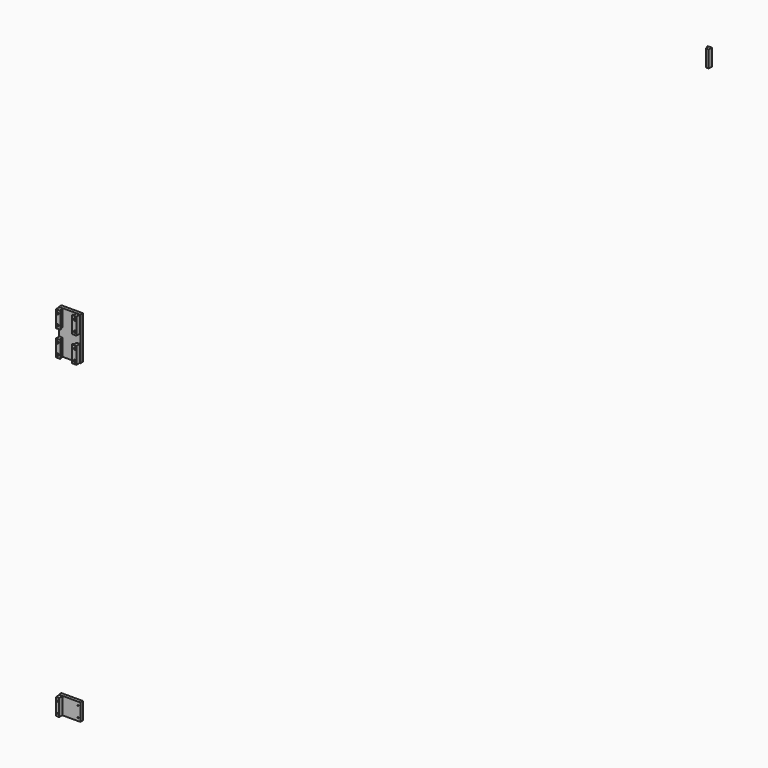
from build123d import *

# Parameters (mm, degrees)
F1_W           = 100
F1_H           = 200
F2_DEPTH       = 15
F3_D           = 5
F4_W           = 15
F4_H           = 78
F4_R           = 2.5
F5_DEPTH       = 20
F7_D           = 6.6
F7_CBORE_D     = 11.25
F7_CBORE_DEPTH = 6
F8_W           = 5
F8_H           = 78
F9_DEPTH       = 5
F10_W          = 100
F10_H          = 80
F11_DEPTH      = 15
F12_W          = 15
F12_H          = 78
F13_DEPTH      = 20
F15_D          = 5
F15_2_D        = 5
F23_DEPTH      = 78


# Not quite as in the source:
# - a pattern or mirror of a feature is missing from the dataset's text; its kind, count and spacing are read off the source's solid


with BuildPart() as f2:
    # F1 (on Front) → F2 (new body)
    with BuildSketch(Plane.XZ):
        with Locations((-2997.1325380377, -2081.9933028066)):
            Rectangle(F1_W, F1_H)
    extrude(amount=F2_DEPTH)

    # F3 (through all)
    with Locations(Plane(origin=(0, 0, 0), x_dir=(1, 0, 0), z_dir=(0, 1, 0))):
        with Locations((-3037.6325380377, 1996.9933028066), (-2956.6325380377, 1996.9933028066), (-2956.6325380377, 2046.9933028066), (-3037.6325380377, 2046.9933028066), (-3037.6325380377, 2116.9933028066), (-2956.6325380377, 2116.9933028066), (-3037.6325380377, 2166.9933028066), (-2956.6325380377, 2166.9933028066)):
            Hole(F3_D / 2)


with BuildPart() as f5:
    # F4 (on face) → F5 (new body)
    with BuildSketch(Plane.XZ.offset(15)):
        with Locations((-3037.1325380377, -2021.9933028066)):
            Rectangle(F4_W, F4_H)
        with Locations((-3037.6325380377, -2046.9933028066)):
            Circle(F4_R, mode=Mode.SUBTRACT)
        with Locations((-3037.6325380377, -1996.9933028066)):
            Circle(F4_R, mode=Mode.SUBTRACT)
    extrude(amount=F5_DEPTH)

    # F7 (through all)
    with Locations(Plane.XZ.offset(35)):
        with Locations((-3037.6325380377, -1996.9933028066), (-3037.6325380377, -2046.9933028066)):
            CounterBoreHole(F7_D / 2, F7_CBORE_D / 2, F7_CBORE_DEPTH)

    # F8 (on face) → F9 (join)
    with BuildSketch(Plane.YZ.offset(-3029.6325380377)):
        with Locations((-32.5, -2021.9933028066)):
            Rectangle(F8_W, F8_H)
    extrude(amount=F9_DEPTH)


with BuildPart() as f11:
    # F10 (on face) → F11 (new body)
    with BuildSketch(Plane.XZ):
        with Locations((-2997.1325380377, -3614.9933028066)):
            Rectangle(F10_W, F10_H)
    extrude(amount=F11_DEPTH)

    # F15 (through all)
    with Locations(Plane.XZ.offset(35)):
        with Locations((-3037.1325380377, -3590.9933028066), (-3037.1325380377, -3640.9933028066)):
            f15 = Hole(F15_D / 2)

    # F15_copies: F15 across plane
    add(f15.mirror(Plane(origin=(-2997.132538, 0, 0), x_dir=(0, 0, 1), z_dir=(1, 0, 0))), mode=Mode.SUBTRACT)


with BuildPart() as f13:
    # F12 (on face) → F13 (new body)
    with BuildSketch(Plane.XZ.offset(15)):
        with Locations((-3037.1325380377, -3614.9933028066)):
            Rectangle(F12_W, F12_H)
    extrude(amount=F13_DEPTH)

    # F15#2 (through all)
    with Locations(Plane.XZ.offset(35)):
        with Locations((-3037.1325380377, -3590.9933028066), (-3037.1325380377, -3640.9933028066)):
            Hole(F15_2_D / 2)


with BuildPart() as f19_1:
    # F19: instance of F5
    add(f5.part.mirror(Plane(origin=(-2997.1325380377, -7.5, -2081.9933028066), x_dir=(0, -1, 0), z_dir=(-1, 0, 0))))


with BuildPart() as f20_1:
    # F20: instance of F5
    add(f5.part.mirror(Plane(origin=(-2997.1325380377, -7.5, -2081.9933028066), x_dir=(1, 0, 0), z_dir=(0, 0, -1))))


with BuildPart() as f20_2:
    # F20: instance of F19_1
    add(f19_1.part.mirror(Plane(origin=(-2997.1325380377, -7.5, -2081.9933028066), x_dir=(1, 0, 0), z_dir=(0, 0, -1))))


with BuildPart() as f23:
    # F22 (on Top) → F23 (new body)
    with BuildSketch(Plane.XY):
        Polygon((-13.8222467692, -21.6615384615), (-13.8222467692, -26.6830769231), (-11.3607083077, -26.6830769231), (-11.3607083077, -26.1907692308), (-7.9145544615, -26.1907692308), (-7.9145544615, -40.8615384615), (-4.173016, -40.8615384615), (2.1285224615, -40.8615384615), (2.9162147692, -40.8615384615), (2.9162147692, -41.3538461538), (5.8700609231, -41.3538461538), (5.8700609231, -21.6615384615), (4.0977532308, -21.6615384615), (-6.1422467692, -21.6615384615), align=None)
    extrude(amount=F23_DEPTH)


solid = Compound([f2.part, f5.part, f11.part, f13.part, f19_1.part, f20_1.part, f20_2.part, f23.part])
